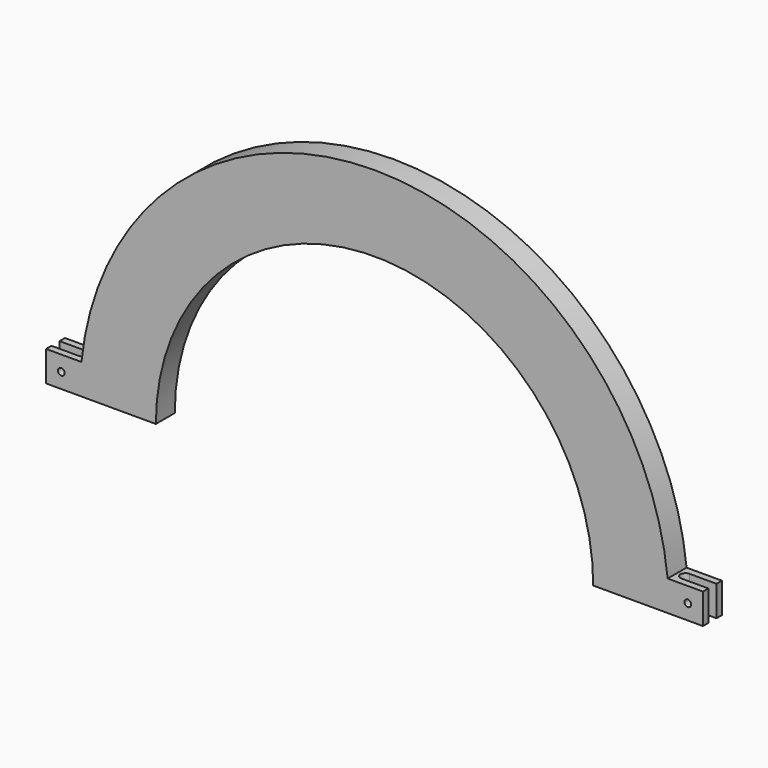
from build123d import *

# Parameters (mm, degrees)
F1_DEPTH = 7
F2_DEPTH = 6
F3_R     = 2
F4_DEPTH = 25
F6_DEPTH = 25


# Not quite as in the source:
# - a pattern or mirror of a feature is missing from the dataset's text; its kind, count and spacing are read off the source's solid


with BuildPart() as f1:
    # F0 (on Front) → F1 (new body, symmetric)
    with BuildSketch(Plane.XZ):
        with BuildLine():
            Line((129.5, 0), (174.5, 0))
            ThreePointArc((174.5, 0), (174.2671322418, 9.0120264206), (173.5691504848, 18))
            ThreePointArc((173.5691504848, 18), (0, 174.5), (-173.5691504848, 18))
            ThreePointArc((-173.5691504848, 18), (-174.2671322418, 9.0120264206), (-174.5, 0))
            Line((-174.5, 0), (-129.5, 0))
            ThreePointArc((-129.5, 0), (0, 129.5), (129.5, 0))
        make_face()
        with BuildLine():
            ThreePointArc((173.5691504848, 18), (174.2671322418, 9.0120264206), (174.5, 0))
            Line((174.5, 0), (194.5, 0))
            Line((194.5, 0), (194.5, 18))
            Line((194.5, 18), (173.5691504848, 18))
        make_face()
        with BuildLine():
            ThreePointArc((-174.5, 0), (-174.2671322418, 9.0120264206), (-173.5691504848, 18))
            Line((-173.5691504848, 18), (-194.5, 18))
            Line((-194.5, 18), (-194.5, 0))
            Line((-194.5, 0), (-174.5, 0))
        make_face()
    extrude(amount=F1_DEPTH, both=True)

    # F0 (on Front) → F2 (join, symmetric)
    with BuildSketch(Plane.XZ):
        with BuildLine():
            Line((129.5, 0), (174.5, 0))
            ThreePointArc((174.5, 0), (174.2671322418, 9.0120264206), (173.5691504848, 18))
            ThreePointArc((173.5691504848, 18), (0, 174.5), (-173.5691504848, 18))
            ThreePointArc((-173.5691504848, 18), (-174.2671322418, 9.0120264206), (-174.5, 0))
            Line((-174.5, 0), (-129.5, 0))
            ThreePointArc((-129.5, 0), (0, 129.5), (129.5, 0))
        make_face()
        with BuildLine():
            ThreePointArc((173.5691504848, 18), (174.2671322418, 9.0120264206), (174.5, 0))
            Line((174.5, 0), (194.5, 0))
            Line((194.5, 0), (194.5, 18))
            Line((194.5, 18), (173.5691504848, 18))
        make_face()
        with BuildLine():
            ThreePointArc((-174.5, 0), (-174.2671322418, 9.0120264206), (-173.5691504848, 18))
            Line((-173.5691504848, 18), (-194.5, 18))
            Line((-194.5, 18), (-194.5, 0))
            Line((-194.5, 0), (-174.5, 0))
        make_face()
    extrude(amount=F2_DEPTH, both=True)

    # F3 (on face) → F4 (cut)
    with BuildSketch(Plane.XZ.offset(7)):
        with Locations((185.5, 9)):
            Circle(F3_R)
    f4 = extrude(amount=-F4_DEPTH, mode=Mode.SUBTRACT)

    # F4_copies: F4 across plane
    add(f4.mirror(Plane(origin=(0, 0, 0), x_dir=(0, 0, -1), z_dir=(-1, 0, 0))), mode=Mode.SUBTRACT)

    # F5 (on face) → F6 (cut)
    with BuildSketch(Plane.XY.offset(18)):
        with BuildLine():
            Line((194.5, 3), (178.5, 3))
            ThreePointArc((178.5, 3), (175.5, 0), (178.5, -3))
            Line((178.5, -3), (194.5, -3))
            Line((194.5, -3), (194.5, 3))
        make_face()
    f6 = extrude(amount=-F6_DEPTH, mode=Mode.SUBTRACT)

    # F6_copies: F6 across plane
    add(f6.mirror(Plane(origin=(0, 0, 0), x_dir=(0, 0, -1), z_dir=(-1, 0, 0))), mode=Mode.SUBTRACT)


solid = f1.part
